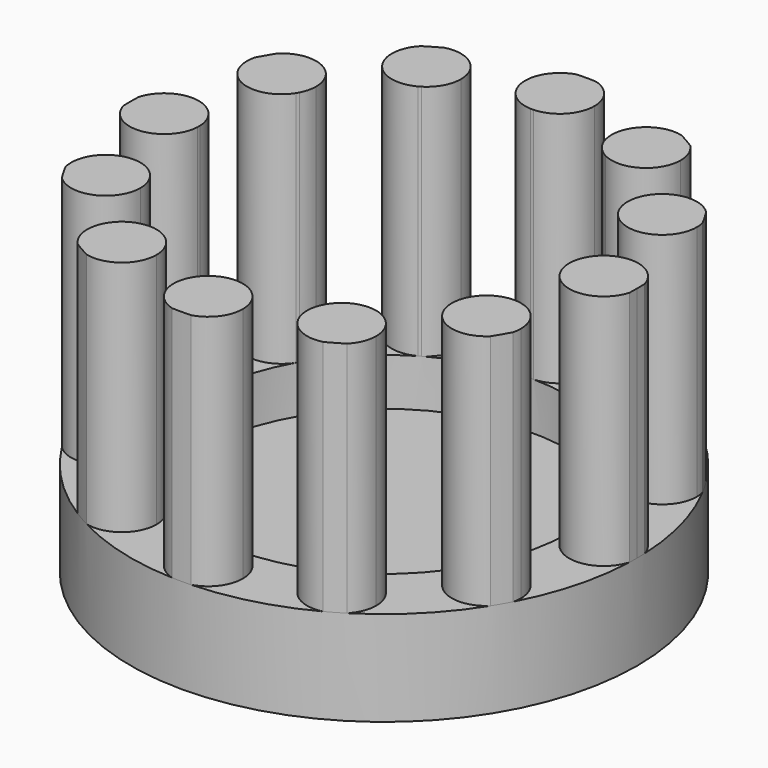
from build123d import *

# Parameters (mm, degrees)
F0_R     = 19.8242320165
F1_DEPTH = 5.08
F0_R_2   = 27.1027644971
F2_DEPTH = 10.16
F4_DEPTH = 25.4


with BuildPart() as f1:
    # F0 (on Top) → F1 (new body)
    with BuildSketch(Plane.XY):
        Circle(F0_R)
    extrude(amount=F1_DEPTH)

    # F0 (on Top) → F2 (join)
    with BuildSketch(Plane.XY):
        Circle(F0_R_2)
        Circle(F0_R, mode=Mode.SUBTRACT)
    extrude(amount=F2_DEPTH)

    # F3 (on face) → F4 (join)
    with BuildSketch(Plane.XY.offset(10.16)):
        with BuildLine():
            ThreePointArc((27.1027644971, 0), (27.0980286069, 0.5066448501), (27.0838225914, 1.0131126398))
            ThreePointArc((27.0838225914, 1.0131126398), (23.0888262615, 3.676897102), (19.823615331, 0.1563657619))
            ThreePointArc((19.823615331, 0.1563657619), (19.8240778445, 0.078183489), (19.8242320165, 0))
            ThreePointArc((19.8242320165, 0), (19.8240778445, -0.078183489), (19.823615331, -0.1563657619))
            ThreePointArc((19.823615331, -0.1563657619), (23.0888262615, -3.676897102), (27.0838225914, -1.0131126398))
            ThreePointArc((27.0838225914, -1.0131126398), (27.0980286069, -0.5066448501), (27.1027644971, 0))
        make_face()
        with BuildLine():
            ThreePointArc((24.0736841586, 11.7613608018), (24.0456154002, 12.2163951196), (23.9618347156, 12.6645300128))
            ThreePointArc((23.9618347156, 12.6645300128), (23.4716825672, 13.5513822485), (22.9487220759, 14.4192925786))
            ThreePointArc((22.9487220759, 14.4192925786), (18.157061535, 14.7286994282), (17.0895715906, 10.0472243876))
            ThreePointArc((17.0895715906, 10.0472243876), (17.1682885368, 9.9121160082), (17.2459373524, 9.7763909435))
            ThreePointArc((17.2459373524, 9.7763909435), (21.404850558, 8.206145204), (24.0736841586, 11.7613608018))
        make_face()
        with BuildLine():
            ThreePointArc((22.9487220759, -14.4192925786), (23.4716825672, -13.5513822485), (23.9618347156, -12.6645300128))
            ThreePointArc((23.9618347156, -12.6645300128), (24.0456154002, -12.2163951196), (24.0736841586, -11.7613608018))
            ThreePointArc((24.0736841586, -11.7613608018), (21.404850558, -8.206145204), (17.2459373524, -9.7763909435))
            ThreePointArc((17.2459373524, -9.7763909435), (17.1682885368, -9.9121160082), (17.0895715906, -10.0472243876))
            ThreePointArc((17.0895715906, -10.0472243876), (18.157061535, -14.7286994282), (22.9487220759, -14.4192925786))
        make_face()
        with BuildLine():
            ThreePointArc((15.4637704856, 20.3712744748), (15.1927300486, 21.7617932839), (14.4192925786, 22.9487220759))
            ThreePointArc((14.4192925786, 22.9487220759), (13.5513822485, 23.4716825672), (12.6645300128, 23.9618347156))
            ThreePointArc((12.6645300128, 23.9618347156), (8.3601268333, 21.833958637), (9.7763909435, 17.2459373524))
            ThreePointArc((9.7763909435, 17.2459373524), (9.9121160082, 17.1682885368), (10.0472243876, 17.0895715906))
            ThreePointArc((10.0472243876, 17.0895715906), (13.6798761402, 17.2047090858), (15.4637704856, 20.3712744748))
        make_face()
        with BuildLine():
            ThreePointArc((12.6645300128, -23.9618347156), (13.5513822485, -23.4716825672), (14.4192925786, -22.9487220759))
            ThreePointArc((14.4192925786, -22.9487220759), (15.1927300486, -21.7617932839), (15.4637704856, -20.3712744748))
            ThreePointArc((15.4637704856, -20.3712744748), (13.6798761402, -17.2047090858), (10.0472243876, -17.0895715906))
            ThreePointArc((10.0472243876, -17.0895715906), (9.9121160082, -17.1682885368), (9.7763909435, -17.2459373524))
            ThreePointArc((9.7763909435, -17.2459373524), (8.3601268333, -21.833958637), (12.6645300128, -23.9618347156))
        make_face()
        with BuildLine():
            ThreePointArc((3.7024096838, 23.5227216035), (2.9545554247, 25.7539633451), (1.0131126398, 27.0838225914))
            ThreePointArc((1.0131126398, 27.0838225914), (0, 27.1027644971), (-1.0131126398, 27.0838225914))
            ThreePointArc((-1.0131126398, 27.0838225914), (-3.676897102, 23.0888262615), (-0.1563657619, 19.823615331))
            ThreePointArc((-0.1563657619, 19.823615331), (0, 19.8242320165), (0.1563657619, 19.823615331))
            ThreePointArc((0.1563657619, 19.823615331), (2.6727109437, 20.9606026215), (3.7024096838, 23.5227216035))
        make_face()
        with BuildLine():
            ThreePointArc((-1.0131126398, -27.0838225914), (0, -27.1027644971), (1.0131126398, -27.0838225914))
            ThreePointArc((1.0131126398, -27.0838225914), (2.9545554247, -25.7539633451), (3.7024096838, -23.5227216035))
            ThreePointArc((3.7024096838, -23.5227216035), (2.6727109437, -20.9606026215), (0.1563657619, -19.823615331))
            ThreePointArc((0.1563657619, -19.823615331), (0, -19.8242320165), (-0.1563657619, -19.823615331))
            ThreePointArc((-0.1563657619, -19.823615331), (-3.676897102, -23.0888262615), (-1.0131126398, -27.0838225914))
        make_face()
        with BuildLine():
            ThreePointArc((-8.0589511179, 20.3712744748), (-9.4849672688, 23.2911837114), (-12.6645300128, 23.9618347156))
            ThreePointArc((-12.6645300128, 23.9618347156), (-13.5513822485, 23.4716825672), (-14.4192925786, 22.9487220759))
            ThreePointArc((-14.4192925786, 22.9487220759), (-14.7286994282, 18.157061535), (-10.0472243876, 17.0895715906))
            ThreePointArc((-10.0472243876, 17.0895715906), (-9.9121160082, 17.1682885368), (-9.7763909435, 17.2459373524))
            ThreePointArc((-9.7763909435, 17.2459373524), (-8.5165950866, 18.5882060743), (-8.0589511179, 20.3712744748))
        make_face()
        with BuildLine():
            ThreePointArc((-14.4192925786, -22.9487220759), (-13.5513822485, -23.4716825672), (-12.6645300128, -23.9618347156))
            ThreePointArc((-12.6645300128, -23.9618347156), (-9.4849672688, -23.2911837114), (-8.0589511179, -20.3712744748))
            ThreePointArc((-8.0589511179, -20.3712744748), (-8.5165950866, -18.5882060743), (-9.7763909435, -17.2459373524))
            ThreePointArc((-9.7763909435, -17.2459373524), (-9.9121160082, -17.1682885368), (-10.0472243876, -17.0895715906))
            ThreePointArc((-10.0472243876, -17.0895715906), (-14.7286994282, -18.157061535), (-14.4192925786, -22.9487220759))
        make_face()
        with BuildLine():
            ThreePointArc((-16.668864791, 11.7613608018), (-18.9281752909, 15.1709505443), (-22.9487220759, 14.4192925786))
            ThreePointArc((-22.9487220759, 14.4192925786), (-23.4716825672, 13.5513822485), (-23.9618347156, 12.6645300128))
            ThreePointArc((-23.9618347156, 12.6645300128), (-21.833958637, 8.3601268333), (-17.2459373524, 9.7763909435))
            ThreePointArc((-17.2459373524, 9.7763909435), (-17.1682885368, 9.9121160082), (-17.0895715906, 10.0472243876))
            ThreePointArc((-17.0895715906, 10.0472243876), (-16.7755794095, 10.8788561477), (-16.668864791, 11.7613608018))
        make_face()
        with BuildLine():
            ThreePointArc((-23.9618347156, -12.6645300128), (-23.4716825672, -13.5513822485), (-22.9487220759, -14.4192925786))
            ThreePointArc((-22.9487220759, -14.4192925786), (-18.9281752909, -15.1709505443), (-16.668864791, -11.7613608018))
            ThreePointArc((-16.668864791, -11.7613608018), (-16.7755794095, -10.8788561477), (-17.0895715906, -10.0472243876))
            ThreePointArc((-17.0895715906, -10.0472243876), (-17.1682885368, -9.9121160082), (-17.2459373524, -9.7763909435))
            ThreePointArc((-17.2459373524, -9.7763909435), (-21.833958637, -8.3601268333), (-23.9618347156, -12.6645300128))
        make_face()
        with BuildLine():
            ThreePointArc((-19.823615331, 0.1563657619), (-23.0888262615, 3.676897102), (-27.0838225914, 1.0131126398))
            ThreePointArc((-27.0838225914, 1.0131126398), (-27.1027644971, 0), (-27.0838225914, -1.0131126398))
            ThreePointArc((-27.0838225914, -1.0131126398), (-23.0888262615, -3.676897102), (-19.823615331, -0.1563657619))
            ThreePointArc((-19.823615331, -0.1563657619), (-19.8242320165, 0), (-19.823615331, 0.1563657619))
        make_face()
    extrude(amount=F4_DEPTH)


solid = f1.part
